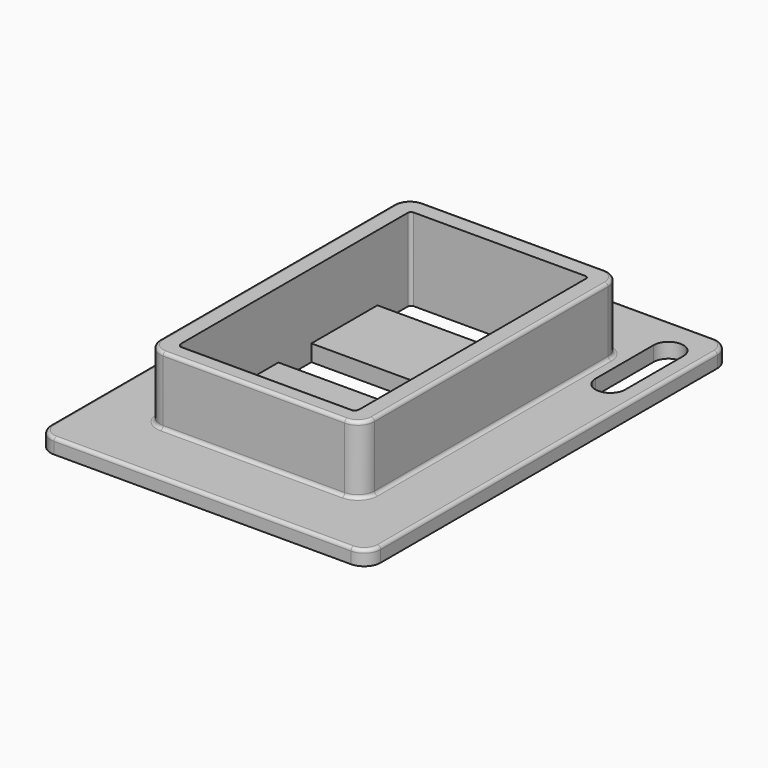
from build123d import *

# Parameters (mm, degrees)
F0_W         = 33.02
F0_H         = 50.038
F0_W_2       = 27.432
F0_H_2       = 44.45
F1_DEPTH     = 12.7
F0_W_3       = 50.8
F0_H_3       = 69.85
F2_DEPTH     = 2.286
F3_W         = 27.432
F3_H         = 12.7
F4_DEPTH     = 2.54
F5_R         = 2.54
F6_R         = 2.54
F7_T1_DEPTH  = 64.77
F7_T3_DEPTH  = 44.958
F7_T5_DEPTH  = 27.432
F7_T7_DEPTH  = 45.72
F7_T9_DEPTH  = 27.94
F7_T12_ANGLE = 90
F7_T14_ANGLE = 90
F7_T16_ANGLE = 90
F7_T18_ANGLE = 90
F7_T20_ANGLE = 90
F7_T22_ANGLE = 90
F7_T24_ANGLE = 90
F7_T26_ANGLE = 90
F7_T27_DEPTH = 44.958
F7_T29_DEPTH = 27.94
F7_T31_DEPTH = 12.7
F7_T33_DEPTH = 12.192
F7_T36_ANGLE = 90
F7_T38_ANGLE = 90
F7_T40_ANGLE = 90
F7_T42_ANGLE = 90
F7_T46_ANGLE = 233.2969892374
F7_T51_ANGLE = 233.2969892374
F10_DEPTH    = 2.287


# Not quite as in the source:
# - a fillet or chamfer that OpenCascade refuses, or shapes differently, is made with other operations: its cross-section is extruded or revolved along the edge and cut away or added
# - two fillets or chamfers of one size are made in one step


with BuildPart() as f1:
    # F0 (on Top) → F1 (new body)
    with BuildSketch(Plane.XY):
        with Locations((-13.8195358872, -22.5519042432)):
            Rectangle(F0_W, F0_H)
        with Locations((-13.8195358872, -22.5519042432)):
            Rectangle(F0_W_2, F0_H_2, mode=Mode.SUBTRACT)
    extrude(amount=F1_DEPTH)

    # F0 (on Top) → F2 (join)
    with BuildSketch(Plane.XY):
        with Locations((-13.8195358872, -22.5519042432)):
            Rectangle(F0_W_3, F0_H_3)
        with Locations((-13.8195358872, -22.5519042432)):
            Rectangle(F0_W, F0_H, mode=Mode.SUBTRACT)
    extrude(amount=F2_DEPTH)

    # F5
    f5_edges = [f1.edges().sort_by_distance(p)[0] for p in [
        (2.690464, 2.467096, 7.493),
        (2.690464, -47.570904, 7.493),
        (-30.329536, 2.467096, 7.493),
        (-30.329536, -47.570904, 7.493),
    ]]
    fillet(f5_edges, radius=F5_R)

    # F6
    f6_edges = [f1.edges().sort_by_distance(p)[0] for p in [
        (11.580464, 12.373096, 1.143),
        (11.580464, -57.476904, 1.143),
        (-39.219536, -57.476904, 1.143),
        (-39.219536, 12.373096, 1.143),
    ]]
    fillet(f6_edges, radius=F6_R)

    # F7: fillet of radius 0.508 on 29 edges, made by hand

    # F7_s2 → F7_t1 (cut)
    with BuildSketch(Plane.XZ.offset(-9.8330957568)):
        with BuildLine():
            ThreePointArc((-38.7115358872, 2.286), (-39.0707461321, 2.1372102448), (-39.2195358872, 1.778))
            Line((-39.2195358872, 1.778), (-39.2195358872, 2.286))
            Line((-39.2195358872, 2.286), (-38.7115358872, 2.286))
        make_face()
        with BuildLine():
            ThreePointArc((11.0724641128, 2.286), (11.4316743576, 2.1372102448), (11.5804641128, 1.778))
            Line((11.5804641128, 1.778), (11.5804641128, 2.286))
            Line((11.5804641128, 2.286), (11.0724641128, 2.286))
        make_face()
    extrude(amount=F7_T1_DEPTH, mode=Mode.SUBTRACT)

    # F7_s4 → F7_t3 (cut)
    with BuildSketch(Plane.XZ.offset(0.0729042432)):
        with BuildLine():
            ThreePointArc((2.6904641128, 12.192), (2.5416743576, 12.5512102448), (2.1824641128, 12.7))
            Line((2.1824641128, 12.7), (2.6904641128, 12.7))
            Line((2.6904641128, 12.7), (2.6904641128, 12.192))
        make_face()
        with BuildLine():
            ThreePointArc((-30.3295358872, 12.192), (-30.1807461321, 12.5512102448), (-29.8215358872, 12.7))
            Line((-29.8215358872, 12.7), (-30.3295358872, 12.7))
            Line((-30.3295358872, 12.7), (-30.3295358872, 12.192))
        make_face()
    extrude(amount=F7_T3_DEPTH, mode=Mode.SUBTRACT)

    # F7_s6 → F7_t5 (cut)
    with BuildSketch(Plane.YZ.offset(-27.5355358872)):
        with BuildLine():
            ThreePointArc((-45.2849042432, 12.7), (-44.9256939984, 12.5512102448), (-44.7769042432, 12.192))
            Line((-44.7769042432, 12.192), (-44.7769042432, 12.7))
            Line((-44.7769042432, 12.7), (-45.2849042432, 12.7))
        make_face()
    extrude(amount=F7_T5_DEPTH, mode=Mode.SUBTRACT)

    # F7_s8 → F7_t7 (cut)
    with BuildSketch(Plane.YZ.offset(-36.6795358872)):
        with BuildLine():
            ThreePointArc((11.8650957568, 2.286), (12.2243060016, 2.1372102448), (12.3730957568, 1.778))
            Line((12.3730957568, 1.778), (12.3730957568, 2.286))
            Line((12.3730957568, 2.286), (11.8650957568, 2.286))
        make_face()
        with BuildLine():
            ThreePointArc((-56.9689042432, 2.286), (-57.3281144881, 2.1372102448), (-57.4769042432, 1.778))
            Line((-57.4769042432, 1.778), (-57.4769042432, 2.286))
            Line((-57.4769042432, 2.286), (-56.9689042432, 2.286))
        make_face()
    extrude(amount=F7_T7_DEPTH, mode=Mode.SUBTRACT)

    # F7_s10 → F7_t9 (cut)
    with BuildSketch(Plane.YZ.offset(-27.7895358872)):
        with BuildLine():
            ThreePointArc((2.4670957568, 12.192), (2.3183060016, 12.5512102448), (1.9590957568, 12.7))
            Line((1.9590957568, 12.7), (2.4670957568, 12.7))
            Line((2.4670957568, 12.7), (2.4670957568, 12.192))
        make_face()
        with BuildLine():
            ThreePointArc((-47.5709042432, 12.192), (-47.4221144881, 12.5512102448), (-47.0629042432, 12.7))
            Line((-47.0629042432, 12.7), (-47.5709042432, 12.7))
            Line((-47.5709042432, 12.7), (-47.5709042432, 12.192))
        make_face()
    extrude(amount=F7_T9_DEPTH, mode=Mode.SUBTRACT)

    # F7_s11 → F7_t12 (revolve, cut)
    with BuildSketch(Plane.XZ.offset(-9.8330957568)):
        with BuildLine():
            ThreePointArc((-38.7115358872, 2.286), (-39.0707461321, 2.1372102448), (-39.2195358872, 1.778))
            Line((-39.2195358872, 1.778), (-39.2195358872, 2.286))
            Line((-39.2195358872, 2.286), (-38.7115358872, 2.286))
        make_face()
    revolve(axis=Axis((-36.6795358872, 9.8330957568, 2.286), (0, 0, -1)), revolution_arc=F7_T12_ANGLE, mode=Mode.SUBTRACT)

    # F7_s13 → F7_t14 (revolve, cut)
    with BuildSketch(Plane.XZ.offset(54.9369042432)):
        with BuildLine():
            ThreePointArc((-38.7115358872, 2.286), (-39.0707461321, 2.1372102448), (-39.2195358872, 1.778))
            Line((-39.2195358872, 1.778), (-39.2195358872, 2.286))
            Line((-39.2195358872, 2.286), (-38.7115358872, 2.286))
        make_face()
    revolve(axis=Axis((-36.6795358872, -54.9369042432, 2.286), (0, 0, 1)), revolution_arc=F7_T14_ANGLE, mode=Mode.SUBTRACT)

    # F7_s15 → F7_t16 (revolve, cut)
    with BuildSketch(Plane.XZ.offset(-9.8330957568)):
        with BuildLine():
            ThreePointArc((11.0724641128, 2.286), (11.4316743576, 2.1372102448), (11.5804641128, 1.778))
            Line((11.5804641128, 1.778), (11.5804641128, 2.286))
            Line((11.5804641128, 2.286), (11.0724641128, 2.286))
        make_face()
    revolve(axis=Axis((9.0404641128, 9.8330957568, 2.286), (0, 0, 1)), revolution_arc=F7_T16_ANGLE, mode=Mode.SUBTRACT)

    # F7_s17 → F7_t18 (revolve, cut)
    with BuildSketch(Plane.YZ.offset(9.0404641128)):
        with BuildLine():
            ThreePointArc((-56.9689042432, 2.286), (-57.3281144881, 2.1372102448), (-57.4769042432, 1.778))
            Line((-57.4769042432, 1.778), (-57.4769042432, 2.286))
            Line((-57.4769042432, 2.286), (-56.9689042432, 2.286))
        make_face()
    revolve(axis=Axis((9.0404641128, -54.9369042432, 2.286), (0, 0, 1)), revolution_arc=F7_T18_ANGLE, mode=Mode.SUBTRACT)

    # F7_s19 → F7_t20 (revolve, cut)
    with BuildSketch(Plane.YZ.offset(0.1504641128)):
        with BuildLine():
            ThreePointArc((2.4670957568, 12.192), (2.3183060016, 12.5512102448), (1.9590957568, 12.7))
            Line((1.9590957568, 12.7), (2.4670957568, 12.7))
            Line((2.4670957568, 12.7), (2.4670957568, 12.192))
        make_face()
    revolve(axis=Axis((0.1504641128, -0.0729042432, 12.7), (0, 0, -1)), revolution_arc=F7_T20_ANGLE, mode=Mode.SUBTRACT)

    # F7_s21 → F7_t22 (revolve, cut)
    with BuildSketch(Plane.XZ.offset(45.0309042432)):
        with BuildLine():
            ThreePointArc((2.6904641128, 12.192), (2.5416743576, 12.5512102448), (2.1824641128, 12.7))
            Line((2.1824641128, 12.7), (2.6904641128, 12.7))
            Line((2.6904641128, 12.7), (2.6904641128, 12.192))
        make_face()
    revolve(axis=Axis((0.1504641128, -45.0309042432, 12.7), (0, 0, -1)), revolution_arc=F7_T22_ANGLE, mode=Mode.SUBTRACT)

    # F7_s23 → F7_t24 (revolve, cut)
    with BuildSketch(Plane.YZ.offset(-27.7895358872)):
        with BuildLine():
            ThreePointArc((2.4670957568, 12.192), (2.3183060016, 12.5512102448), (1.9590957568, 12.7))
            Line((1.9590957568, 12.7), (2.4670957568, 12.7))
            Line((2.4670957568, 12.7), (2.4670957568, 12.192))
        make_face()
    revolve(axis=Axis((-27.7895358872, -0.0729042432, 12.7), (0, 0, 1)), revolution_arc=F7_T24_ANGLE, mode=Mode.SUBTRACT)

    # F7_s25 → F7_t26 (revolve, cut)
    with BuildSketch(Plane.XZ.offset(45.0309042432)):
        with BuildLine():
            ThreePointArc((-30.3295358872, 12.192), (-30.1807461321, 12.5512102448), (-29.8215358872, 12.7))
            Line((-29.8215358872, 12.7), (-30.3295358872, 12.7))
            Line((-30.3295358872, 12.7), (-30.3295358872, 12.192))
        make_face()
    revolve(axis=Axis((-27.7895358872, -45.0309042432, 12.7), (0, 0, 1)), revolution_arc=F7_T26_ANGLE, mode=Mode.SUBTRACT)

    # F7_s28 → F7_t27 (join)
    with BuildSketch(Plane.XZ.offset(0.0729042432)):
        with BuildLine():
            ThreePointArc((-30.8375358872, 2.286), (-30.4783256424, 2.4347897552), (-30.3295358872, 2.794))
            Line((-30.3295358872, 2.794), (-30.3295358872, 2.286))
            Line((-30.3295358872, 2.286), (-30.8375358872, 2.286))
        make_face()
        with BuildLine():
            ThreePointArc((3.1984641128, 2.286), (2.8392538679, 2.4347897552), (2.6904641128, 2.794))
            Line((2.6904641128, 2.794), (2.6904641128, 2.286))
            Line((2.6904641128, 2.286), (3.1984641128, 2.286))
        make_face()
    extrude(amount=F7_T27_DEPTH)

    # F7_s30 → F7_t29 (join)
    with BuildSketch(Plane.YZ.offset(-27.7895358872)):
        with BuildLine():
            ThreePointArc((2.9750957568, 2.286), (2.6158855119, 2.4347897552), (2.4670957568, 2.794))
            Line((2.4670957568, 2.794), (2.4670957568, 2.286))
            Line((2.4670957568, 2.286), (2.9750957568, 2.286))
        make_face()
        with BuildLine():
            ThreePointArc((-48.0789042432, 2.286), (-47.7196939984, 2.4347897552), (-47.5709042432, 2.794))
            Line((-47.5709042432, 2.794), (-47.5709042432, 2.286))
            Line((-47.5709042432, 2.286), (-48.0789042432, 2.286))
        make_face()
    extrude(amount=F7_T29_DEPTH)

    # F7_s32 → F7_t31 (join)
    with BuildSketch(Plane.XY):
        with BuildLine():
            ThreePointArc((-0.1035358872, -0.8349042432), (-0.2523256424, -0.4756939984), (-0.6115358872, -0.3269042432))
            Line((-0.6115358872, -0.3269042432), (-0.1035358872, -0.3269042432))
            Line((-0.1035358872, -0.3269042432), (-0.1035358872, -0.8349042432))
        make_face()
        with BuildLine():
            ThreePointArc((-27.5355358872, -0.8349042432), (-27.3867461321, -0.4756939984), (-27.0275358872, -0.3269042432))
            Line((-27.0275358872, -0.3269042432), (-27.5355358872, -0.3269042432))
            Line((-27.5355358872, -0.3269042432), (-27.5355358872, -0.8349042432))
        make_face()
    extrude(amount=F7_T31_DEPTH)

    # F7_s34 → F7_t33 (join)
    with BuildSketch(Plane.XY):
        with BuildLine():
            ThreePointArc((-0.6115358872, -44.7769042432), (-0.2523256424, -44.6281144881), (-0.1035358872, -44.2689042432))
            Line((-0.1035358872, -44.2689042432), (-0.1035358872, -44.7769042432))
            Line((-0.1035358872, -44.7769042432), (-0.6115358872, -44.7769042432))
        make_face()
        with BuildLine():
            ThreePointArc((-27.5355358872, -44.2689042432), (-27.3867461321, -44.6281144881), (-27.0275358872, -44.7769042432))
            Line((-27.0275358872, -44.7769042432), (-27.5355358872, -44.7769042432))
            Line((-27.5355358872, -44.7769042432), (-27.5355358872, -44.2689042432))
        make_face()
    extrude(amount=F7_T33_DEPTH)

    # F7_s35 → F7_t36 (revolve)
    with BuildSketch(Plane.YZ.offset(0.1504641128)):
        with BuildLine():
            ThreePointArc((2.9750957568, 2.286), (2.6158855119, 2.4347897552), (2.4670957568, 2.794))
            Line((2.4670957568, 2.794), (2.4670957568, 2.286))
            Line((2.4670957568, 2.286), (2.9750957568, 2.286))
        make_face()
    revolve(axis=Axis((0.1504641128, -0.0729042432, 2.286), (0, 0, -1)), revolution_arc=F7_T36_ANGLE)

    # F7_s37 → F7_t38 (revolve)
    with BuildSketch(Plane.XZ.offset(45.0309042432)):
        with BuildLine():
            ThreePointArc((3.1984641128, 2.286), (2.8392538679, 2.4347897552), (2.6904641128, 2.794))
            Line((2.6904641128, 2.794), (2.6904641128, 2.286))
            Line((2.6904641128, 2.286), (3.1984641128, 2.286))
        make_face()
    revolve(axis=Axis((0.1504641128, -45.0309042432, 2.286), (0, 0, -1)), revolution_arc=F7_T38_ANGLE)

    # F7_s39 → F7_t40 (revolve)
    with BuildSketch(Plane.YZ.offset(-27.7895358872)):
        with BuildLine():
            ThreePointArc((2.9750957568, 2.286), (2.6158855119, 2.4347897552), (2.4670957568, 2.794))
            Line((2.4670957568, 2.794), (2.4670957568, 2.286))
            Line((2.4670957568, 2.286), (2.9750957568, 2.286))
        make_face()
    revolve(axis=Axis((-27.7895358872, -0.0729042432, 2.286), (0, 0, 1)), revolution_arc=F7_T40_ANGLE)

    # F7_s41 → F7_t42 (revolve)
    with BuildSketch(Plane.XZ.offset(45.0309042432)):
        with BuildLine():
            ThreePointArc((-30.8375358872, 2.286), (-30.4783256424, 2.4347897552), (-30.3295358872, 2.794))
            Line((-30.3295358872, 2.794), (-30.3295358872, 2.286))
            Line((-30.3295358872, 2.286), (-30.8375358872, 2.286))
        make_face()
    revolve(axis=Axis((-27.7895358872, -45.0309042432, 2.286), (0, 0, 1)), revolution_arc=F7_T42_ANGLE)


with BuildPart() as f4:
    # F3 (on face) → F4 (new body)
    with BuildSketch(Plane(origin=(0, 0, 0), x_dir=(1, 0, 0), z_dir=(0, 0, -1))):
        with Locations((-13.8195358872, 32.0769042432)):
            Rectangle(F3_W, F3_H)
    extrude(amount=-F4_DEPTH)


with BuildPart() as f4b:
    # F3 (on face) → F4, piece 2 (new body)
    with BuildSketch(Plane(origin=(0, 0, 0), x_dir=(1, 0, 0), z_dir=(0, 0, -1))):
        with Locations((-13.8195358872, 13.0269042432)):
            Rectangle(F3_W, F3_H)
    extrude(amount=-F4_DEPTH)


with BuildPart() as f7_tool44:
    # F7_s45 → F7_t46 (revolve)
    with BuildSketch(Plane(origin=(0, -34.9509742358, 26.0545104015), x_dir=(1, 0, 0), z_dir=(0, 0.8017442393, -0.5976672776))):
        with BuildLine():
            ThreePointArc((-27.5355358872, 18.3064396714), (-27.3867461321, 17.9472294266), (-27.0275358872, 17.7984396714))
            Line((-27.0275358872, 17.7984396714), (-27.5355358872, 17.7984396714))
            Line((-27.5355358872, 17.7984396714), (-27.5355358872, 18.3064396714))
        make_face()
    revolve(axis=Axis((-27.5355358872, -45.2849042432, 12.192), (-1, 0, 0)), revolution_arc=F7_T46_ANGLE)

    split(bisect_by=Plane.XY.offset(12.7), keep=Keep.BOTTOM)


with BuildPart() as f1_1:
    add(f1.part)

    # F7_t43: union F7_tool44
    add(f7_tool44.part)


with BuildPart() as f7_tool49:
    # F7_s50 → F7_t51 (revolve)
    with BuildSketch(Plane(origin=(0, -34.9509742358, 26.0545104015), x_dir=(1, 0, 0), z_dir=(0, 0.8017442393, -0.5976672776))):
        with BuildLine():
            ThreePointArc((-0.6115358872, 17.7984396714), (-0.2523256424, 17.9472294266), (-0.1035358872, 18.3064396714))
            Line((-0.1035358872, 18.3064396714), (-0.1035358872, 17.7984396714))
            Line((-0.1035358872, 17.7984396714), (-0.6115358872, 17.7984396714))
        make_face()
    revolve(axis=Axis((-0.1035358872, -45.2849042432, 12.192), (-1, 0, 0)), revolution_arc=F7_T51_ANGLE)

    split(bisect_by=Plane.XY.offset(12.7), keep=Keep.BOTTOM)


with BuildPart() as f1_2:
    add(f1_1.part)

    # F7_t48: union F7_tool49
    add(f7_tool49.part)

    # F9 (on face) → F10 (cut, through all)
    with BuildSketch(Plane.XY.offset(2.286)):
        with BuildLine():
            ThreePointArc((9.1306788937, 6.3603448817), (6.8446788937, 8.6463448817), (4.5586788937, 6.3603448817))
            Line((4.5586788937, 6.3603448817), (4.5586788937, -4.8249972189))
            ThreePointArc((4.5586788937, -4.8249972189), (6.8446788937, -7.1109972189), (9.1306788937, -4.8249972189))
            Line((9.1306788937, -4.8249972189), (9.1306788937, 6.3603448817))
        make_face()
    extrude(amount=-F10_DEPTH, mode=Mode.SUBTRACT)


solid = Compound([f4.part, f4b.part, f1_2.part])
